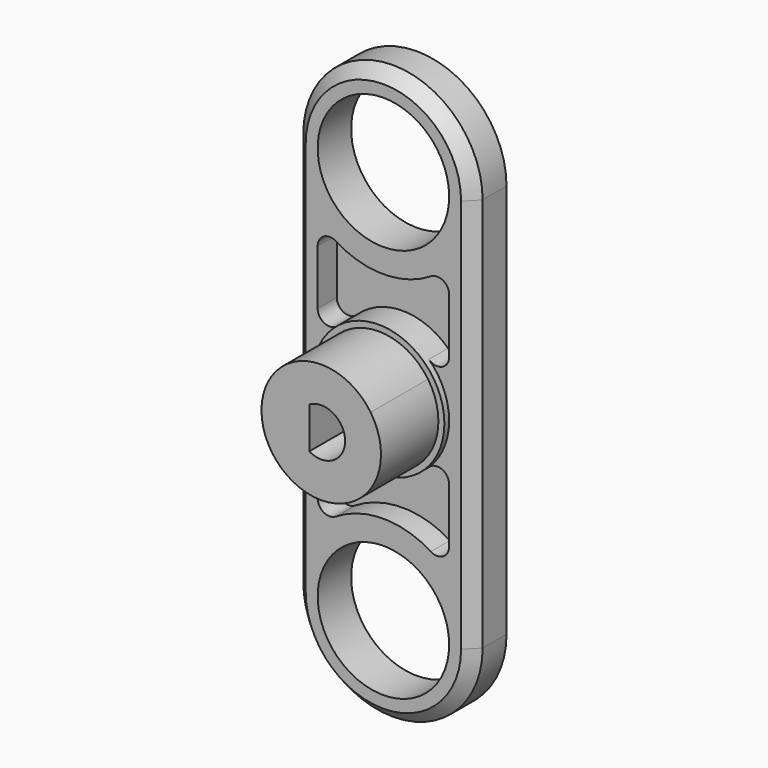
from build123d import *

# Parameters (mm, degrees)
F0_R          = 11
F1_DEPTH      = 7
F2_DEPTH      = 20
F3_DEPTH      = 3
F3_DEPTH_BACK = 12.5
F4_DEPTH      = 3
F5_R          = 2
F6_DEPTH      = 5.5
F8_DEPTH      = 8
F9_SIZE       = 2


# Not quite as in the source:
# - a fillet or chamfer that OpenCascade refuses, or shapes differently, is made with other operations: its cross-section is extruded or revolved along the edge and cut away or added


with BuildPart() as f1:
    # F0 (on Front) → F1 (new body)
    with BuildSketch(Plane.XZ):
        with BuildLine():
            ThreePointArc((11, 22.8019609728), (13.9642400438, 27.5227744249), (15, 33))
            ThreePointArc((15, 33), (0, 48), (-15, 33))
            ThreePointArc((-15, 33), (-13.9642400438, 27.5227744249), (-11, 22.8019609728))
            ThreePointArc((-11, 22.8019609728), (0, 18), (11, 22.8019609728))
        make_face()
        with Locations((0, 33)):
            Circle(F0_R, mode=Mode.SUBTRACT)
        with BuildLine():
            ThreePointArc((-15, -33), (0, -48), (15, -33))
            ThreePointArc((15, -33), (13.9642400438, -27.5227744249), (11, -22.8019609728))
            ThreePointArc((11, -22.8019609728), (0, -18), (-11, -22.8019609728))
            ThreePointArc((-11, -22.8019609728), (-13.9642400438, -27.5227744249), (-15, -33))
        make_face()
        with Locations((0, -33)):
            Circle(F0_R, mode=Mode.SUBTRACT)
        with BuildLine():
            ThreePointArc((-11, 22.8019609728), (-13.9642400438, 27.5227744249), (-15, 33))
            Line((-15, 33), (-15, -33))
            ThreePointArc((-15, -33), (-13.9642400438, -27.5227744249), (-11, -22.8019609728))
            Line((-11, -22.8019609728), (-11, -9.3808315196))
            ThreePointArc((-11, -9.3808315196), (-9.7844645406, -7.5410990976), (-7.6153846154, -7.9376266705))
            ThreePointArc((-7.6153846154, -7.9376266705), (-11, 0), (-7.6153846154, 7.9376266705))
            ThreePointArc((-7.6153846154, 7.9376266705), (-9.7844645406, 7.5410990976), (-11, 9.3808315196))
            Line((-11, 9.3808315196), (-11, 22.8019609728))
        make_face()
        with BuildLine():
            Line((15, -33), (15, 33))
            ThreePointArc((15, 33), (13.9642400438, 27.5227744249), (11, 22.8019609728))
            Line((11, 22.8019609728), (11, 9.3808315196))
            ThreePointArc((11, 9.3808315196), (9.7844645406, 7.5410990976), (7.6153846154, 7.9376266705))
            ThreePointArc((7.6153846154, 7.9376266705), (10.1185283211, 4.314554973), (11, 0))
            ThreePointArc((11, 0), (10.1185283211, -4.314554973), (7.6153846154, -7.9376266705))
            ThreePointArc((7.6153846154, -7.9376266705), (9.7844645406, -7.5410990976), (11, -9.3808315196))
            Line((11, -9.3808315196), (11, -22.8019609728))
            ThreePointArc((11, -22.8019609728), (13.9642400438, -27.5227744249), (15, -33))
        make_face()
        with BuildLine():
            ThreePointArc((11, 0), (10.1185283211, 4.314554973), (7.6153846154, 7.9376266705))
            ThreePointArc((7.6153846154, 7.9376266705), (0, 11), (-7.6153846154, 7.9376266705))
            ThreePointArc((-7.6153846154, 7.9376266705), (-11, 0), (-7.6153846154, -7.9376266705))
            ThreePointArc((-7.6153846154, -7.9376266705), (0, -11), (7.6153846154, -7.9376266705))
            ThreePointArc((7.6153846154, -7.9376266705), (10.1185283211, -4.314554973), (11, 0))
        make_face()
        with BuildLine():
            ThreePointArc((-8.2567722168, 5.6414282376), (0, 10), (8.2567722168, 5.6414282376))
            ThreePointArc((8.2567722168, 5.6414282376), (10, 0), (8.2567722168, -5.6414282376))
            ThreePointArc((8.2567722168, -5.6414282376), (0, -10), (-8.2567722168, -5.6414282376))
            ThreePointArc((-8.2567722168, -5.6414282376), (-10, 0), (-8.2567722168, 5.6414282376))
        make_face(mode=Mode.SUBTRACT)
        with BuildLine():
            ThreePointArc((8.2567722168, -5.6414282376), (10, 0), (8.2567722168, 5.6414282376))
            ThreePointArc((8.2567722168, 5.6414282376), (0, 10), (-8.2567722168, 5.6414282376))
            ThreePointArc((-8.2567722168, 5.6414282376), (-10, 0), (-8.2567722168, -5.6414282376))
            ThreePointArc((-8.2567722168, -5.6414282376), (0, -10), (8.2567722168, -5.6414282376))
        make_face()
        with BuildLine():
            ThreePointArc((-2, 3.4641016151), (2, 3.4641016151), (4, 0))
            ThreePointArc((4, 0), (2, -3.4641016151), (-2, -3.4641016151))
            ThreePointArc((-2, -3.4641016151), (-4, 0), (-2, 3.4641016151))
        make_face(mode=Mode.SUBTRACT)
        with BuildLine():
            Line((-2, -3.4641016151), (-2, 3.4641016151))
            ThreePointArc((-2, 3.4641016151), (-4, 0), (-2, -3.4641016151))
        make_face()
        with BuildLine():
            ThreePointArc((-2, -3.4641016151), (2, -3.4641016151), (4, 0))
            ThreePointArc((4, 0), (2, 3.4641016151), (-2, 3.4641016151))
            Line((-2, 3.4641016151), (-2, -3.4641016151))
        make_face()
    extrude(amount=F1_DEPTH)

    # F0 (on Front) → F2 (join)
    with BuildSketch(Plane.XZ):
        with BuildLine():
            ThreePointArc((8.2567722168, -5.6414282376), (10, 0), (8.2567722168, 5.6414282376))
            ThreePointArc((8.2567722168, 5.6414282376), (0, 10), (-8.2567722168, 5.6414282376))
            ThreePointArc((-8.2567722168, 5.6414282376), (-10, 0), (-8.2567722168, -5.6414282376))
            ThreePointArc((-8.2567722168, -5.6414282376), (0, -10), (8.2567722168, -5.6414282376))
        make_face()
        with BuildLine():
            ThreePointArc((-2, 3.4641016151), (2, 3.4641016151), (4, 0))
            ThreePointArc((4, 0), (2, -3.4641016151), (-2, -3.4641016151))
            ThreePointArc((-2, -3.4641016151), (-4, 0), (-2, 3.4641016151))
        make_face(mode=Mode.SUBTRACT)
        with BuildLine():
            Line((-2, -3.4641016151), (-2, 3.4641016151))
            ThreePointArc((-2, 3.4641016151), (-4, 0), (-2, -3.4641016151))
        make_face()
    extrude(amount=F2_DEPTH)

    # F0 (on Front) → F3 (join, two sides)
    with BuildSketch(Plane.XZ) as f3_sk:
        with BuildLine():
            Line((-2, -3.4641016151), (-2, 3.4641016151))
            ThreePointArc((-2, 3.4641016151), (-4, 0), (-2, -3.4641016151))
        make_face()
        with BuildLine():
            ThreePointArc((-2, -3.4641016151), (2, -3.4641016151), (4, 0))
            ThreePointArc((4, 0), (2, 3.4641016151), (-2, 3.4641016151))
            Line((-2, 3.4641016151), (-2, -3.4641016151))
        make_face()
    extrude(amount=F3_DEPTH)
    extrude(f3_sk.sketch, amount=-F3_DEPTH_BACK)

    # F0 (on Front) → F4 (join)
    with BuildSketch(Plane.XZ):
        with BuildLine():
            Line((11, 9.3808315196), (11, 22.8019609728))
            ThreePointArc((11, 22.8019609728), (0, 18), (-11, 22.8019609728))
            Line((-11, 22.8019609728), (-11, 9.3808315196))
            ThreePointArc((-11, 9.3808315196), (-9.7844645406, 7.5410990976), (-7.6153846154, 7.9376266705))
            ThreePointArc((-7.6153846154, 7.9376266705), (0, 11), (7.6153846154, 7.9376266705))
            ThreePointArc((7.6153846154, 7.9376266705), (9.7844645406, 7.5410990976), (11, 9.3808315196))
        make_face()
        with BuildLine():
            ThreePointArc((-11, -22.8019609728), (0, -18), (11, -22.8019609728))
            Line((11, -22.8019609728), (11, -9.3808315196))
            ThreePointArc((11, -9.3808315196), (9.7844645406, -7.5410990976), (7.6153846154, -7.9376266705))
            ThreePointArc((7.6153846154, -7.9376266705), (0, -11), (-7.6153846154, -7.9376266705))
            ThreePointArc((-7.6153846154, -7.9376266705), (-9.7844645406, -7.5410990976), (-11, -9.3808315196))
            Line((-11, -9.3808315196), (-11, -22.8019609728))
        make_face()
        with BuildLine():
            ThreePointArc((11, 0), (10.1185283211, 4.314554973), (7.6153846154, 7.9376266705))
            ThreePointArc((7.6153846154, 7.9376266705), (0, 11), (-7.6153846154, 7.9376266705))
            ThreePointArc((-7.6153846154, 7.9376266705), (-11, 0), (-7.6153846154, -7.9376266705))
            ThreePointArc((-7.6153846154, -7.9376266705), (0, -11), (7.6153846154, -7.9376266705))
            ThreePointArc((7.6153846154, -7.9376266705), (10.1185283211, -4.314554973), (11, 0))
        make_face()
        with BuildLine():
            ThreePointArc((-8.2567722168, 5.6414282376), (0, 10), (8.2567722168, 5.6414282376))
            ThreePointArc((8.2567722168, 5.6414282376), (10, 0), (8.2567722168, -5.6414282376))
            ThreePointArc((8.2567722168, -5.6414282376), (0, -10), (-8.2567722168, -5.6414282376))
            ThreePointArc((-8.2567722168, -5.6414282376), (-10, 0), (-8.2567722168, 5.6414282376))
        make_face(mode=Mode.SUBTRACT)
    extrude(amount=F4_DEPTH)

    # F5
    f5_edges = [f1.edges().sort_by_distance(p)[0] for p in [
        (-11, -5, -22.801961),
        (11, -5, -22.801961),
        (11, -5, 22.801961),
        (-11, -5, 22.801961),
    ]]
    fillet(f5_edges, radius=F5_R)

    # F0 (on Front) → F6 (join)
    with BuildSketch(Plane.XZ):
        with BuildLine():
            ThreePointArc((11, 0), (10.1185283211, 4.314554973), (7.6153846154, 7.9376266705))
            ThreePointArc((7.6153846154, 7.9376266705), (0, 11), (-7.6153846154, 7.9376266705))
            ThreePointArc((-7.6153846154, 7.9376266705), (-11, 0), (-7.6153846154, -7.9376266705))
            ThreePointArc((-7.6153846154, -7.9376266705), (0, -11), (7.6153846154, -7.9376266705))
            ThreePointArc((7.6153846154, -7.9376266705), (10.1185283211, -4.314554973), (11, 0))
        make_face()
        with BuildLine():
            ThreePointArc((-8.2567722168, 5.6414282376), (0, 10), (8.2567722168, 5.6414282376))
            ThreePointArc((8.2567722168, 5.6414282376), (10, 0), (8.2567722168, -5.6414282376))
            ThreePointArc((8.2567722168, -5.6414282376), (0, -10), (-8.2567722168, -5.6414282376))
            ThreePointArc((-8.2567722168, -5.6414282376), (-10, 0), (-8.2567722168, 5.6414282376))
        make_face(mode=Mode.SUBTRACT)
        with BuildLine():
            ThreePointArc((8.2567722168, -5.6414282376), (10, 0), (8.2567722168, 5.6414282376))
            ThreePointArc((8.2567722168, 5.6414282376), (0, 10), (-8.2567722168, 5.6414282376))
            ThreePointArc((-8.2567722168, 5.6414282376), (-10, 0), (-8.2567722168, -5.6414282376))
            ThreePointArc((-8.2567722168, -5.6414282376), (0, -10), (8.2567722168, -5.6414282376))
        make_face()
        with BuildLine():
            ThreePointArc((-2, 3.4641016151), (2, 3.4641016151), (4, 0))
            ThreePointArc((4, 0), (2, -3.4641016151), (-2, -3.4641016151))
            ThreePointArc((-2, -3.4641016151), (-4, 0), (-2, 3.4641016151))
        make_face(mode=Mode.SUBTRACT)
    extrude(amount=-F6_DEPTH)

    # F7: chamfer of 5.5 x 6 on 1 edges, made by hand


with BuildPart() as f7_tool2:
    # F7_s3 → F7_t4 (revolve)
    with BuildSketch(Plane(origin=(0, 0, 0), x_dir=(0, 1, 0), z_dir=(0.7216024246, 0, 0.6923076923))):
        Polygon((0, 11), (5.5, 5), (5.5, 11), align=None)
    revolve(axis=Axis((0, 5.5, 0), (0, -1, 0)))

    split(bisect_by=Plane.XZ, keep=Keep.BOTTOM)


with BuildPart() as f1_1:
    add(f1.part)

    # F7_t1: cut F7_tool2
    add(f7_tool2.part, mode=Mode.SUBTRACT)

    # F0 (on Front) → F8 (join)
    with BuildSketch(Plane.XZ):
        with BuildLine():
            ThreePointArc((11, 0), (10.1185283211, 4.314554973), (7.6153846154, 7.9376266705))
            ThreePointArc((7.6153846154, 7.9376266705), (0, 11), (-7.6153846154, 7.9376266705))
            ThreePointArc((-7.6153846154, 7.9376266705), (-11, 0), (-7.6153846154, -7.9376266705))
            ThreePointArc((-7.6153846154, -7.9376266705), (0, -11), (7.6153846154, -7.9376266705))
            ThreePointArc((7.6153846154, -7.9376266705), (10.1185283211, -4.314554973), (11, 0))
        make_face()
        with BuildLine():
            ThreePointArc((-8.2567722168, 5.6414282376), (0, 10), (8.2567722168, 5.6414282376))
            ThreePointArc((8.2567722168, 5.6414282376), (10, 0), (8.2567722168, -5.6414282376))
            ThreePointArc((8.2567722168, -5.6414282376), (0, -10), (-8.2567722168, -5.6414282376))
            ThreePointArc((-8.2567722168, -5.6414282376), (-10, 0), (-8.2567722168, 5.6414282376))
        make_face(mode=Mode.SUBTRACT)
    extrude(amount=F8_DEPTH)

    # F9
    f9_edges = [f1_1.edges().sort_by_distance(p)[0] for p in [
        (0, -7, 48),
        (15, -7, 0),
        (-15, -7, 0),
        (0, -7, -48),
    ]]
    chamfer(f9_edges, length=F9_SIZE)


solid = f1_1.part
